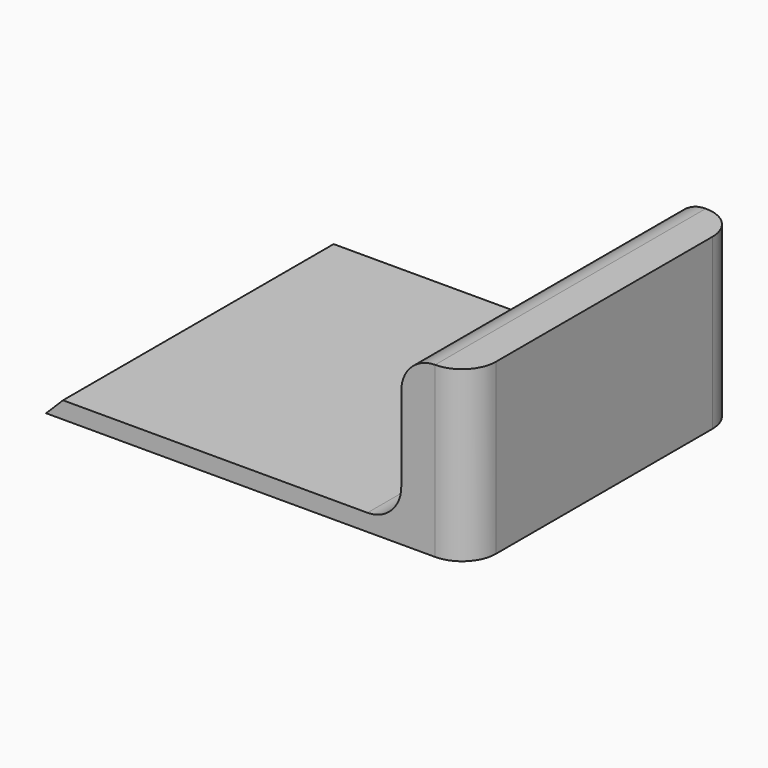
from build123d import *

# Parameters (mm, degrees)
F1_DEPTH = 10
F2_R     = 0.99999


# Not quite as in the source:
# - a fillet or chamfer is up to 0.001 mm smaller than in the source, because OpenCascade refuses the exact size


with BuildPart() as f1:
    # F0 (on Front) → F1 (new body)
    with BuildSketch(Plane.XZ):
        Polygon((0.5, 0.5), (0, 0), (12.5, 0), (12.5, 5), (10.5, 5), (10.5, 0.5), align=None)
    extrude(amount=F1_DEPTH)

    # F2 (radius 1 in the source; OpenCascade refuses exactly that, so slightly less here)
    f2_edges = [f1.edges().sort_by_distance(p)[0] for p in [
        (10.5, -5, 0.5),
        (12.5, -10, 2.5),
        (12.5, 0, 2.5),
        (10.5, -5, 5),
    ]]
    fillet(f2_edges, radius=F2_R)


solid = f1.part
